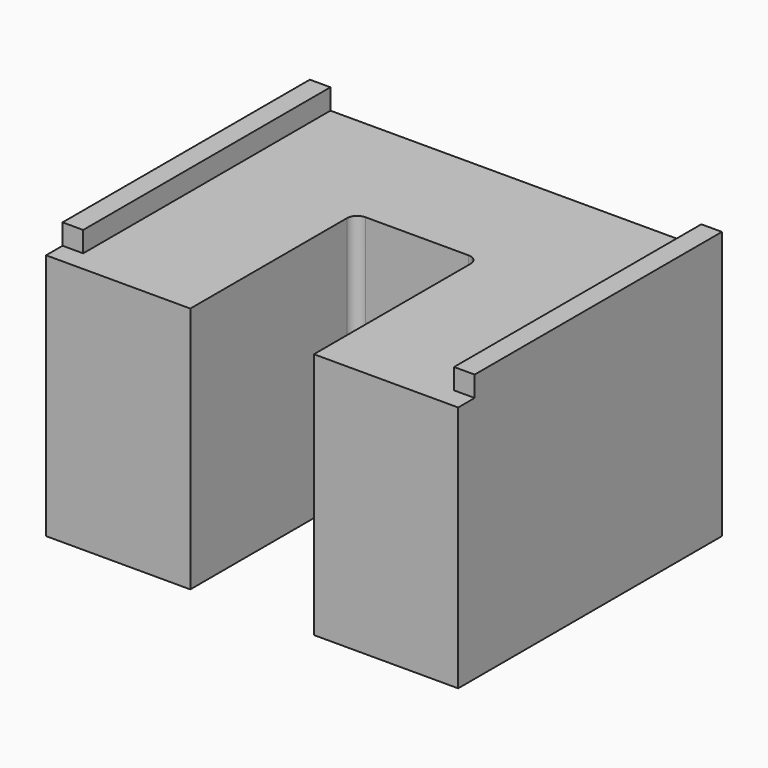
from build123d import *

# Parameters (mm, degrees)
F1_DEPTH = 120
F4_W     = 10
F4_H     = 10
F5_DEPTH = 150
F6_D     = 9
F6_DEPTH = 15
F6_TIP   = 2.7038727856
F7_R     = 5


# Not quite as in the source:
# - a feature names something its author has since deleted; it is built from what else it names


with BuildPart() as f1:
    # F0 (on Top) → F1 (new body)
    with BuildSketch(Plane.XY):
        Polygon((100, -80), (100, 80), (-100, 80), (-100, -80), (-55, -80), (-30, -80), (-30, -10), (-30, 20), (30, 20), (30, -16.3740634173), (30, -80), (55, -80), align=None)
    extrude(amount=F1_DEPTH)

    # F4 (on face) → F5 (join)
    with BuildSketch(Plane(origin=(0, 80, 0), x_dir=(-1, 0, 0), z_dir=(0, 1, 0))):
        with Locations((95, 125)):
            Rectangle(F4_W, F4_H)
        with Locations((-95, 125)):
            Rectangle(F4_W, F4_H)
    extrude(amount=-F5_DEPTH)

    # F6
    with Locations(Plane(origin=(0, 0, 0), x_dir=(1, 0, 0), z_dir=(0, 0, -1))):
        with Locations((-80, -60), (-80, 60), (80, 60), (80, -60)):
            Hole(F6_D / 2, depth=F6_DEPTH)
            with Locations((0, 0, -(F6_DEPTH + F6_TIP / 2))):  # 118° drill point
                Cone(0, F6_D / 2, F6_TIP, mode=Mode.SUBTRACT)

    # F7
    f7_edges = [f1.edges().sort_by_distance(p)[0] for p in [
        (-30, 20, 60),
        (30, 20, 60),
    ]]
    fillet(f7_edges, radius=F7_R)


solid = f1.part
